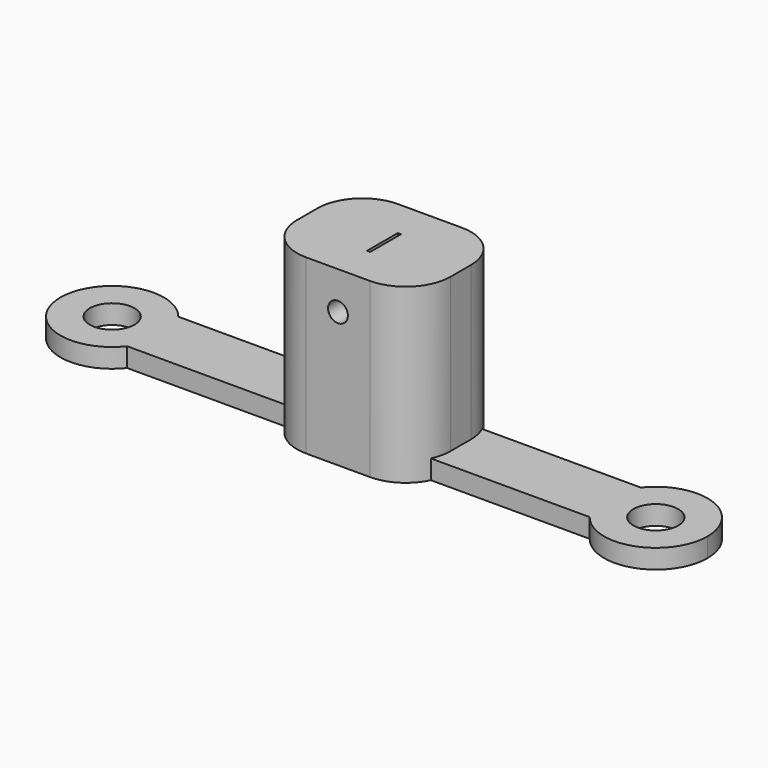
from build123d import *

# Parameters (mm, degrees)
F1_DEPTH     = 3
F3_D         = 7
F4_W         = 24
F4_H         = 18
F5_DEPTH     = 27
F6_R         = 1.55
F7_DEPTH     = 12.5
F8_R         = 1.75
F9_DEPTH     = 12
F10_R        = 4
F11_DEPTH    = 3.4
F12_T4_DEPTH = 62
F12_T9_DEPTH = 62
F13_R        = 7
F14_T4_DEPTH = 62
F14_T9_DEPTH = 62
F15_R        = 7
F16_W        = 0.5
F16_H        = 6
F17_DEPTH    = 20
F18_R        = 5
F19_DEPTH    = 10
F20_R        = 3
F20_R_2      = 1.55
F21_DEPTH    = 3


# Not quite as in the source:
# - a fillet or chamfer that OpenCascade refuses, or shapes differently, is made with other operations: its cross-section is extruded or revolved along the edge and cut away or added


with BuildPart() as f1:
    # F0 (on Top) → F1 (new body)
    with BuildSketch(Plane.XY):
        with BuildLine():
            Line((42.5, 5), (42.5, -5))
            Line((42.5, -5), (36.1522351233, -5))
            ThreePointArc((36.1522351233, -5), (45.1458596679, -7.635020992), (50.5804776424, 0))
            ThreePointArc((50.5804776424, 0), (45.1458596679, 7.635020992), (36.1522351233, 5))
            Line((36.1522351233, 5), (42.5, 5))
        make_face()
        with BuildLine():
            ThreePointArc((-36.1522351233, 5), (-50.5804776424, 0), (-36.1522351233, -5))
            Line((-36.1522351233, -5), (-42.5, -5))
            Line((-42.5, -5), (-42.5, 5))
            Line((-42.5, 5), (-36.1522351233, 5))
        make_face()
        with BuildLine():
            Line((36.1522351233, -5), (42.5, -5))
            Line((42.5, -5), (42.5, 5))
            Line((42.5, 5), (36.1522351233, 5))
            ThreePointArc((36.1522351233, 5), (34.4195223576, 0), (36.1522351233, -5))
        make_face()
        with BuildLine():
            Line((-36.1522351233, -5), (36.1522351233, -5))
            ThreePointArc((36.1522351233, -5), (34.4195223576, 0), (36.1522351233, 5))
            Line((36.1522351233, 5), (-36.1522351233, 5))
            ThreePointArc((-36.1522351233, 5), (-34.864979008, 2.6458596679), (-34.4195223576, 0))
            ThreePointArc((-34.4195223576, 0), (-34.864979008, -2.6458596679), (-36.1522351233, -5))
        make_face()
        with BuildLine():
            Line((-42.5, -5), (-36.1522351233, -5))
            ThreePointArc((-36.1522351233, -5), (-34.864979008, -2.6458596679), (-34.4195223576, 0))
            ThreePointArc((-34.4195223576, 0), (-34.864979008, 2.6458596679), (-36.1522351233, 5))
            Line((-36.1522351233, 5), (-42.5, 5))
            Line((-42.5, 5), (-42.5, -5))
        make_face()
    extrude(amount=F1_DEPTH)

    # F3 (through all)
    with Locations(Plane.XY.offset(3)):
        with Locations((-42.5, 0), (42.5, 0)):
            Hole(F3_D / 2)

    # F4 (on Top) → F5 (join)
    with BuildSketch(Plane.XY):
        Rectangle(F4_W, F4_H)
    extrude(amount=F5_DEPTH)

    # F6 (on Front) → F7 (cut, symmetric)
    with BuildSketch(Plane.XZ):
        with Locations((0, 21.0996698588)):
            Circle(F6_R)
    extrude(amount=F7_DEPTH, both=True, mode=Mode.SUBTRACT)

    # F8 (on face) → F9 (cut)
    with BuildSketch(Plane(origin=(-12, 0, 0), x_dir=(0, -1, 0), z_dir=(-1, 0, 0))):
        with Locations((0, 21.061129868)):
            Circle(F8_R)
    extrude(amount=-F9_DEPTH, mode=Mode.SUBTRACT)

    # F10 (on face) → F11 (cut)
    with BuildSketch(Plane(origin=(-12, 0, 0), x_dir=(0, -1, 0), z_dir=(-1, 0, 0))):
        with Locations((0, 21.061129868)):
            Circle(F10_R)
    extrude(amount=-F11_DEPTH, mode=Mode.SUBTRACT)

    # F12: fillet of radius 7 on 1 edges, made by hand


with BuildPart() as f12_tool2:
    # F12_s3 → F12_t4 (new body)
    with BuildSketch(Plane.XY.offset(-17.5)):
        with BuildLine():
            ThreePointArc((-5, 9), (-9.9497474683, 6.9497474683), (-12, 2))
            Line((-12, 2), (-12, 9))
            Line((-12, 9), (-5, 9))
        make_face()
    extrude(amount=F12_T4_DEPTH)

    split(bisect_by=Plane.XZ.offset(-5), keep=Keep.BOTTOM)


with BuildPart() as f1_1:
    add(f1.part)

    # F12_t1: cut F12_tool2
    add(f12_tool2.part, mode=Mode.SUBTRACT)


with BuildPart() as f12_tool7:
    # F12_s8 → F12_t9 (new body)
    with BuildSketch(Plane.XY.offset(-17.5)):
        with BuildLine():
            ThreePointArc((-5, 9), (-9.9497474683, 6.9497474683), (-12, 2))
            Line((-12, 2), (-12, 9))
            Line((-12, 9), (-5, 9))
        make_face()
    extrude(amount=F12_T9_DEPTH)

    split(bisect_by=Plane.XY.offset(3), keep=Keep.TOP)


with BuildPart() as f1_2:
    add(f1_1.part)

    # F12_t6: cut F12_tool7
    add(f12_tool7.part, mode=Mode.SUBTRACT)

    # F13
    f13_edges = [f1_2.edges().sort_by_distance(p)[0] for p in [
        (12, 9, 13.5),
    ]]
    fillet(f13_edges, radius=F13_R)

    # F14: fillet of radius 7 on 1 edges, made by hand


with BuildPart() as f14_tool2:
    # F14_s3 → F14_t4 (new body)
    with BuildSketch(Plane.XY.offset(-17.5)):
        with BuildLine():
            ThreePointArc((-5, -9), (-9.9497474683, -6.9497474683), (-12, -2))
            Line((-12, -2), (-12, -9))
            Line((-12, -9), (-5, -9))
        make_face()
    extrude(amount=F14_T4_DEPTH)

    split(bisect_by=Plane.XZ.offset(5), keep=Keep.TOP)


with BuildPart() as f1_3:
    add(f1_2.part)

    # F14_t1: cut F14_tool2
    add(f14_tool2.part, mode=Mode.SUBTRACT)


with BuildPart() as f14_tool7:
    # F14_s8 → F14_t9 (new body)
    with BuildSketch(Plane.XY.offset(-17.5)):
        with BuildLine():
            ThreePointArc((-5, -9), (-9.9497474683, -6.9497474683), (-12, -2))
            Line((-12, -2), (-12, -9))
            Line((-12, -9), (-5, -9))
        make_face()
    extrude(amount=F14_T9_DEPTH)

    split(bisect_by=Plane.XY.offset(3), keep=Keep.TOP)


with BuildPart() as f1_4:
    add(f1_3.part)

    # F14_t6: cut F14_tool7
    add(f14_tool7.part, mode=Mode.SUBTRACT)

    # F15
    f15_edges = [f1_4.edges().sort_by_distance(p)[0] for p in [
        (12, -9, 13.5),
    ]]
    fillet(f15_edges, radius=F15_R)

    # F16 (on face) → F17 (cut)
    with BuildSketch(Plane.XY.offset(27)):
        Rectangle(F16_W, F16_H)
    extrude(amount=-F17_DEPTH, mode=Mode.SUBTRACT)

    # F18 (on face) → F19 (cut)
    with BuildSketch(Plane(origin=(0, 0, 0), x_dir=(1, 0, 0), z_dir=(0, 0, -1))):
        Circle(F18_R)
    extrude(amount=-F19_DEPTH, mode=Mode.SUBTRACT)

    # F20 (on face) → F21 (cut)
    with BuildSketch(Plane(origin=(0, 9, 0), x_dir=(-1, 0, 0), z_dir=(0, 1, 0))):
        with Locations((0, 21.0996698588)):
            Circle(F20_R)
        with Locations((0, 21.0996698588)):
            Circle(F20_R_2, mode=Mode.SUBTRACT)
    extrude(amount=-F21_DEPTH, mode=Mode.SUBTRACT)


solid = f1_4.part
